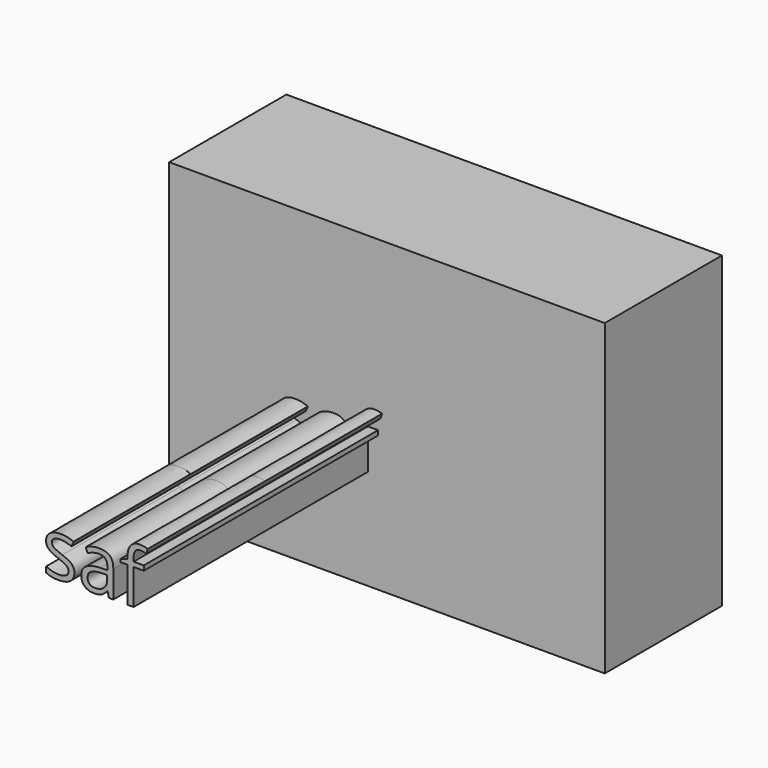
from build123d import *

# Parameters (mm, degrees)
F0_W          = 74.367
F0_H          = 52.665
F1_DEPTH      = 25
F1_DEPTH_BACK = 25
F2_TEXT_SIZE  = 12.7445036776
F3_DEPTH      = 25
F4_DEPTH      = 25


# Not quite as in the source:
# - Text() gives the source's letters only with a copy of the font that has no kerning and outlines rounded to 1/6400 em; it was checked with that copy


with BuildPart() as f1:
    # F0 (on Front) → F1 (new body, two sides)
    with BuildSketch(Plane.XZ) as f1_sk:
        Rectangle(F0_W, F0_H)
    extrude(amount=F1_DEPTH)
    extrude(f1_sk.sketch, amount=-F1_DEPTH_BACK)

    # F2 (on face) → F3 (join)
    with BuildSketch(Plane.XZ.offset(25)):
        with Locations((-18.8598741141, -9.1760426478)):
            Text('saf', F2_TEXT_SIZE, font='Open Sans', text_align=(TextAlign.LEFT, TextAlign.BOTTOM))
    extrude(amount=F3_DEPTH)

    # F4 (cut): a face of the model
    f4_faces = [f1.faces().sort_by_distance(p)[0] for p in [
        (0.1301475619, -25, 0.0756830863),
    ]]
    extrude(f4_faces, amount=-F4_DEPTH, mode=Mode.SUBTRACT)


solid = f1.part
